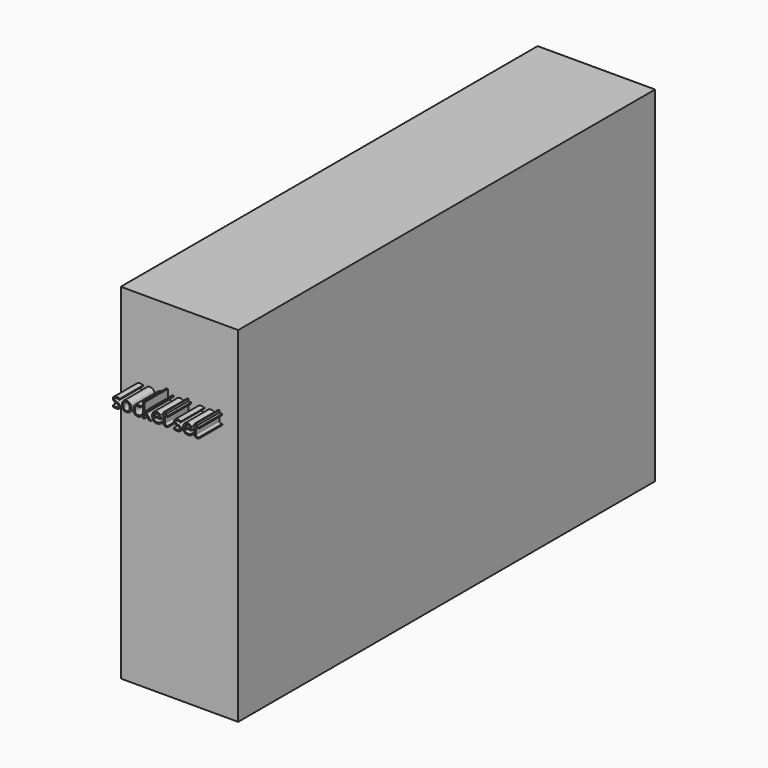
from build123d import *

# Parameters (mm, degrees)
F0_W         = 101.6
F0_H         = 298.45
F1_DEPTH     = 450.85
F2_TEXT_SIZE = 16.244087669
F3_DEPTH     = 25.4


# Not quite as in the source:
# - Text() gives the source's letters only with a copy of the font that has no kerning and outlines rounded to 1/6400 em; it was checked with that copy


with BuildPart() as f1:
    # F0 (on Front) → F1 (new body)
    with BuildSketch(Plane.XZ):
        Rectangle(F0_W, F0_H)
    extrude(amount=F1_DEPTH)

    # F2 (on face) → F3 (join)
    with BuildSketch(Plane.XZ.offset(450.85)):
        with Locations((-38.1, 72.2535880324)):
            Text('socket set', F2_TEXT_SIZE, font='Open Sans', text_align=(TextAlign.LEFT, TextAlign.BOTTOM))
    extrude(amount=F3_DEPTH)


solid = f1.part
